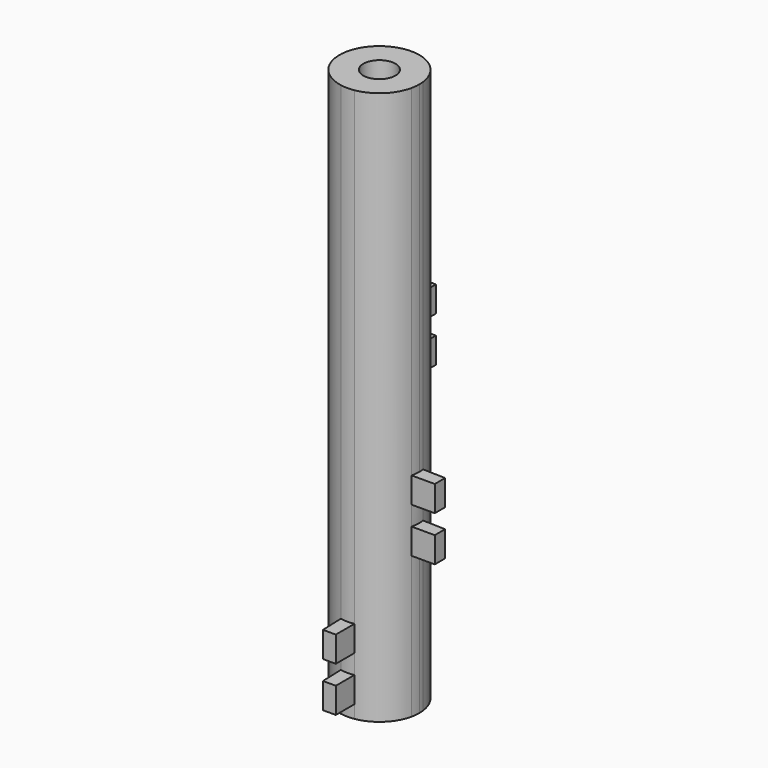
from build123d import *
from build123d import SkipClean  # not in build123d's __all__

# Parameters (mm, degrees)
F0_R      = 3.175
F1_DEPTH  = 127
F2_DEPTH  = 76.2
F3_DEPTH  = 71.12
F4_DEPTH  = 50.8
F5_DEPTH  = 45.72
F6_DEPTH  = 25.4
F7_DEPTH  = 20.32
F9_DEPTH  = 8.89
F10_DEPTH = 3.81
F12_DEPTH = 8.89
F13_DEPTH = 3.81
F15_DEPTH = 8.89
F16_DEPTH = 3.81
F17_DEPTH = 17.78


# Not quite as in the source:
# - after a boolean that leaves OpenCascade's solid faulty, fix() repairs it


with BuildPart() as f1:
    # F0 (on Top) → F1 (new body)
    with BuildSketch(Plane.XY):
        with BuildLine():
            ThreePointArc((7.6934750952, -1.6764), (7.8287386883, -0.8430459954), (7.874, 0))
            ThreePointArc((7.874, 0), (7.8574202107, 0.5107089515), (7.8077506647, 1.0192671673))
            ThreePointArc((7.8077506647, 1.0192671673), (5.6566372636, 5.4774383491), (1.27, 7.7709057387))
            ThreePointArc((1.27, 7.7709057387), (0, 7.874), (-1.27, 7.7709057387))
            ThreePointArc((-1.27, 7.7709057387), (-7.8735779463, 0.0815249862), (-1.430634249, -7.7429426994))
            ThreePointArc((-1.430634249, -7.7429426994), (-0.0815249862, -7.8735779463), (1.27, -7.7709057387))
            ThreePointArc((1.27, -7.7709057387), (5.4195683864, -5.7121059606), (7.6934750952, -1.6764))
        make_face()
        Circle(F0_R, mode=Mode.SUBTRACT)
    extrude(amount=F1_DEPTH)

    # F0 (on Top) → F2 (join)
    with BuildSketch(Plane.XY):
        with BuildLine():
            ThreePointArc((-1.27, 7.7709057387), (0, 7.874), (1.27, 7.7709057387))
            Line((1.27, 7.7709057387), (1.27, 12.3429057387))
            Line((1.27, 12.3429057387), (-1.27, 12.3429057387))
            Line((-1.27, 12.3429057387), (-1.27, 7.7709057387))
        make_face()
    extrude(amount=F2_DEPTH)

    # F0 (on Top) → F3 (cut)
    with BuildSketch(Plane.XY):
        with BuildLine():
            ThreePointArc((-1.27, 7.7709057387), (0, 7.874), (1.27, 7.7709057387))
            Line((1.27, 7.7709057387), (1.27, 12.3429057387))
            Line((1.27, 12.3429057387), (-1.27, 12.3429057387))
            Line((-1.27, 12.3429057387), (-1.27, 7.7709057387))
        make_face()
    with SkipClean():  # cleaning this boolean's faces spoils the solid; the shape is the same uncleaned
        extrude(amount=F3_DEPTH, mode=Mode.SUBTRACT)

    # F0 (on Top) → F4 (join)
    with BuildSketch(Plane.XY):
        with BuildLine():
            ThreePointArc((7.8077506647, 1.0192671673), (7.8574202107, 0.5107089515), (7.874, 0))
            ThreePointArc((7.874, 0), (7.8287386883, -0.8430459954), (7.6934750952, -1.6764))
            Line((7.6934750952, -1.6764), (12.2654750952, -1.6764))
            Line((12.2654750952, -1.6764), (12.2654750952, 0.8636))
            Line((12.2654750952, 0.8636), (7.8077506647, 1.0192671673))
        make_face()
    extrude(amount=F4_DEPTH)

    add(f1.part.fix(), mode=Mode.REPLACE)

    # F0 (on Top) → F5 (cut)
    with BuildSketch(Plane.XY):
        with BuildLine():
            ThreePointArc((7.8077506647, 1.0192671673), (7.8574202107, 0.5107089515), (7.874, 0))
            ThreePointArc((7.874, 0), (7.8287386883, -0.8430459954), (7.6934750952, -1.6764))
            Line((7.6934750952, -1.6764), (12.2654750952, -1.6764))
            Line((12.2654750952, -1.6764), (12.2654750952, 0.8636))
            Line((12.2654750952, 0.8636), (7.8077506647, 1.0192671673))
        make_face()
    with SkipClean():  # cleaning this boolean's faces spoils the solid; the shape is the same uncleaned
        extrude(amount=F5_DEPTH, mode=Mode.SUBTRACT)

    # F0 (on Top) → F6 (join)
    with BuildSketch(Plane.XY):
        with BuildLine():
            Line((1.27, -12.3429057387), (1.27, -7.7709057387))
            ThreePointArc((1.27, -7.7709057387), (-0.0815249862, -7.8735779463), (-1.430634249, -7.7429426994))
            Line((-1.430634249, -7.7429426994), (-1.27, -12.3429057387))
            Line((-1.27, -12.3429057387), (1.27, -12.3429057387))
        make_face()
    extrude(amount=F6_DEPTH)

    add(f1.part.fix(), mode=Mode.REPLACE)

    # F0 (on Top) → F7 (cut)
    with BuildSketch(Plane.XY):
        with BuildLine():
            Line((1.27, -12.3429057387), (1.27, -7.7709057387))
            ThreePointArc((1.27, -7.7709057387), (-0.0815249862, -7.8735779463), (-1.430634249, -7.7429426994))
            Line((-1.430634249, -7.7429426994), (-1.27, -12.3429057387))
            Line((-1.27, -12.3429057387), (1.27, -12.3429057387))
        make_face()
    with SkipClean():  # cleaning this boolean's faces spoils the solid; the shape is the same uncleaned
        extrude(amount=F7_DEPTH, mode=Mode.SUBTRACT)

    # F8 (on face) → F9 (join)
    with BuildSketch(Plane.XY.offset(76.2)):
        with BuildLine():
            Line((1.27, 12.3429057387), (-1.27, 12.3429057387))
            Line((-1.27, 12.3429057387), (-1.27, 7.7709057387))
            ThreePointArc((-1.27, 7.7709057387), (0, 7.874), (1.27, 7.7709057387))
            Line((1.27, 7.7709057387), (1.27, 12.3429057387))
        make_face()
    extrude(amount=F9_DEPTH)

    # F8 (on face) → F10 (cut)
    with BuildSketch(Plane.XY.offset(76.2)):
        with BuildLine():
            Line((1.27, 12.3429057387), (-1.27, 12.3429057387))
            Line((-1.27, 12.3429057387), (-1.27, 7.7709057387))
            ThreePointArc((-1.27, 7.7709057387), (0, 7.874), (1.27, 7.7709057387))
            Line((1.27, 7.7709057387), (1.27, 12.3429057387))
        make_face()
    with SkipClean():  # cleaning this boolean's faces spoils the solid; the shape is the same uncleaned
        extrude(amount=F10_DEPTH, mode=Mode.SUBTRACT)

    # F11 (on face) → F12 (join)
    with BuildSketch(Plane.XY.offset(50.8)):
        with BuildLine():
            Line((12.2654750952, 0.8636), (7.8077506647, 1.0192671673))
            ThreePointArc((7.8077506647, 1.0192671673), (7.8669343066, -0.3334975508), (7.6934750952, -1.6764))
            Line((7.6934750952, -1.6764), (12.2654750952, -1.6764))
            Line((12.2654750952, -1.6764), (12.2654750952, 0.8636))
        make_face()
    extrude(amount=F12_DEPTH)

    # F11 (on face) → F13 (cut)
    with BuildSketch(Plane.XY.offset(50.8)):
        with BuildLine():
            Line((12.2654750952, 0.8636), (7.8077506647, 1.0192671673))
            ThreePointArc((7.8077506647, 1.0192671673), (7.8669343066, -0.3334975508), (7.6934750952, -1.6764))
            Line((7.6934750952, -1.6764), (12.2654750952, -1.6764))
            Line((12.2654750952, -1.6764), (12.2654750952, 0.8636))
        make_face()
    with SkipClean():  # cleaning this boolean's faces spoils the solid; the shape is the same uncleaned
        extrude(amount=F13_DEPTH, mode=Mode.SUBTRACT)

    # F14 (on face) → F15 (join)
    with BuildSketch(Plane.XY.offset(25.4)):
        with BuildLine():
            ThreePointArc((1.27, -7.7709057387), (-0.0815249862, -7.8735779463), (-1.430634249, -7.7429426994))
            Line((-1.430634249, -7.7429426994), (-1.27, -12.3429057387))
            Line((-1.27, -12.3429057387), (1.27, -12.3429057387))
            Line((1.27, -12.3429057387), (1.27, -7.7709057387))
        make_face()
    extrude(amount=F15_DEPTH)

    # F14 (on face) → F16 (cut)
    with BuildSketch(Plane.XY.offset(25.4)):
        with BuildLine():
            ThreePointArc((1.27, -7.7709057387), (-0.0815249862, -7.8735779463), (-1.430634249, -7.7429426994))
            Line((-1.430634249, -7.7429426994), (-1.27, -12.3429057387))
            Line((-1.27, -12.3429057387), (1.27, -12.3429057387))
            Line((1.27, -12.3429057387), (1.27, -7.7709057387))
        make_face()
    extrude(amount=F16_DEPTH, mode=Mode.SUBTRACT)

    # F0 (on Top) → F17 (cut)
    with BuildSketch(Plane.XY):
        with BuildLine():
            ThreePointArc((7.6934750952, -1.6764), (7.8287386883, -0.8430459954), (7.874, 0))
            ThreePointArc((7.874, 0), (7.8574202107, 0.5107089515), (7.8077506647, 1.0192671673))
            ThreePointArc((7.8077506647, 1.0192671673), (5.6566372636, 5.4774383491), (1.27, 7.7709057387))
            ThreePointArc((1.27, 7.7709057387), (0, 7.874), (-1.27, 7.7709057387))
            ThreePointArc((-1.27, 7.7709057387), (-7.8735779463, 0.0815249862), (-1.430634249, -7.7429426994))
            ThreePointArc((-1.430634249, -7.7429426994), (-0.0815249862, -7.8735779463), (1.27, -7.7709057387))
            ThreePointArc((1.27, -7.7709057387), (5.4195683864, -5.7121059606), (7.6934750952, -1.6764))
        make_face()
        Circle(F0_R, mode=Mode.SUBTRACT)
    extrude(amount=F17_DEPTH, mode=Mode.SUBTRACT)


solid = f1.part
